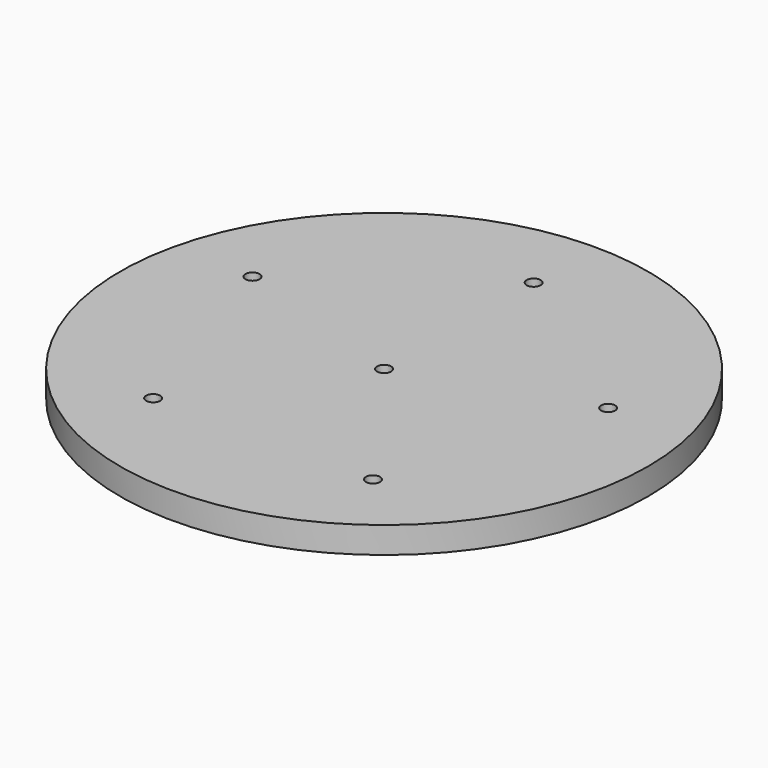
from build123d import *

# Parameters (mm, degrees)
F0_R            = 60
F1_DEPTH        = 6
F3_D            = 3.2
F6_D            = 3.2
F6_COPIES_COUNT = 5


# Not quite as in the source:
# - a pattern or mirror of a feature is missing from the dataset's text; its kind, count and spacing are read off the source's solid


with BuildPart() as f1:
    # F0 (on Top) → F1 (new body)
    with BuildSketch(Plane.XY):
        Circle(F0_R)
    extrude(amount=F1_DEPTH)

    # F3 (through all)
    with Locations(Plane.XY.offset(6)):
        with Locations((0, 0)):
            Hole(F3_D / 2)

    # F6 (through all)
    with Locations(Plane.XY.offset(6)):
        with Locations((0, 42.5)):
            f6 = Hole(F6_D / 2)

    # F6_copies: F6 ×5 about axis
    f6_copies_axis = Axis((0, 0, 0), (0, 0, 1))
    for i in range(1, F6_COPIES_COUNT):
        add(f6.rotate(f6_copies_axis, i * 360 / F6_COPIES_COUNT), mode=Mode.SUBTRACT)


solid = f1.part
